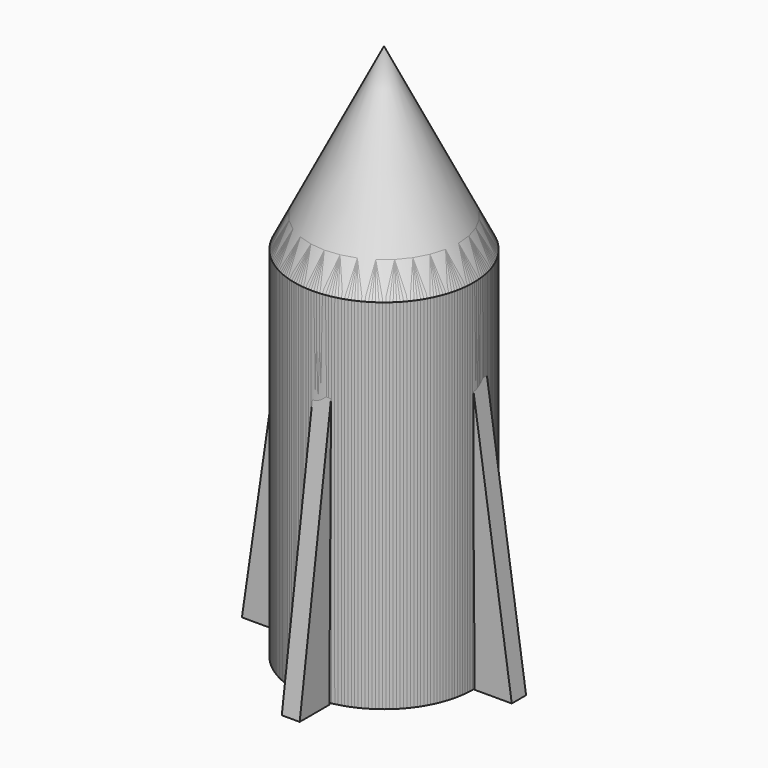
from build123d import *

# Parameters (mm, degrees)
F3_DEPTH = 2.54
F5_COUNT = 4


with BuildPart() as f1:
    # F0 (on Front) → F1 (revolve)
    with BuildSketch(Plane.XZ):
        Polygon((0, 76.2), (0, 0), (12.7, 0), (12.7, 22.9247231036), (12.7, 50.8), align=None)
    revolve(axis=Axis((0, 0, 38.1), (0, 0, -1)))

    # F2 (on Front) → F3 (join)
    with BuildSketch(Plane.XZ):
        Polygon((12.5680267164, 38.0988282072), (12.8668397665, 0), (18.1223098189, 0), align=None)
    extrude(amount=-F3_DEPTH)


with BuildPart() as f5_1:
    # F5: instance of F1
    add(f1.part.rotate(Axis((0, 0, 30.8235287666), (0, 0, 1)), 1 * 360 / F5_COUNT))


with BuildPart() as f5_2:
    # F5: instance of F1
    add(f1.part.rotate(Axis((0, 0, 30.8235287666), (0, 0, 1)), 2 * 360 / F5_COUNT))


with BuildPart() as f5_3:
    # F5: instance of F1
    add(f1.part.rotate(Axis((0, 0, 30.8235287666), (0, 0, 1)), 3 * 360 / F5_COUNT))


solid = Compound([f1.part, f5_1.part, f5_2.part, f5_3.part])
